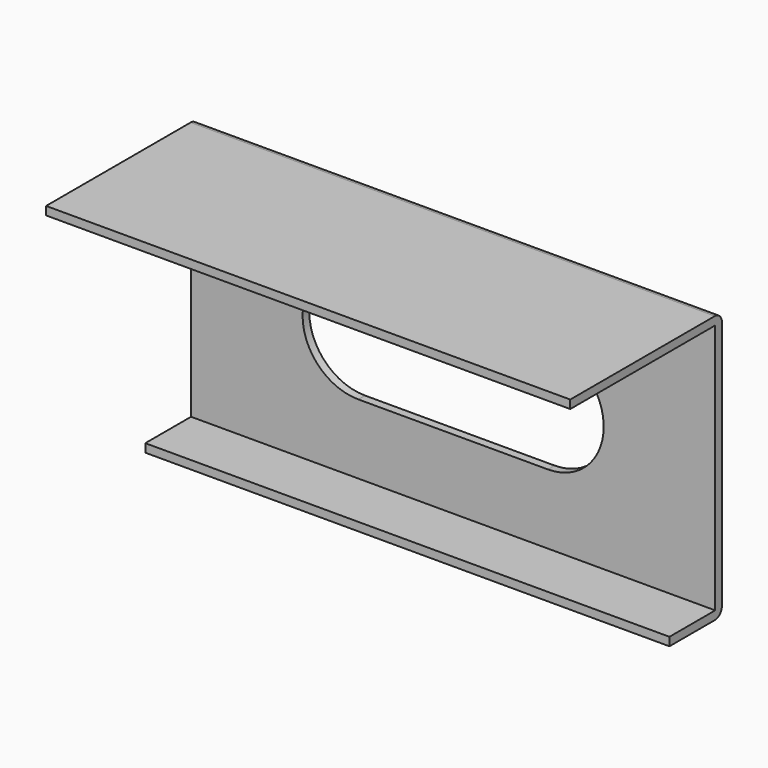
from build123d import *

# Parameters (mm, degrees)
F1_DEPTH = 298.45
F2_R     = 5.08
F4_D     = 63.5
F6_DEPTH = 25.4


with BuildPart() as f1:
    # F0 (on Right) → F1 (new body)
    with BuildSketch(Plane.YZ):
        Polygon((0, -85.7519404639), (0, 66.6480595361), (-107.95, 66.6480595361), (-107.95, 61.8728595361), (-4.7752, 61.8728595361), (-4.7752, -80.9767404639), (-37.338, -80.9767404639), (-37.338, -85.7519404639), align=None)
    extrude(amount=F1_DEPTH)

    # F2
    f2_edges = [f1.edges().sort_by_distance(p)[0] for p in [
        (149.225, 0, 66.64806),
        (149.225, 0, -85.75194),
    ]]
    fillet(f2_edges, radius=F2_R)

    # F4 (through all)
    with Locations(Plane(origin=(0, 0, 0), x_dir=(-1, 0, 0), z_dir=(0, 1, 0))):
        with Locations((-203.2, -9.5519404639), (-95.25, -9.5519404639)):
            Hole(F4_D / 2)

    # F5 (on face) → F6 (cut)
    with BuildSketch(Plane(origin=(0, 0, 0), x_dir=(-1, 0, 0), z_dir=(0, 1, 0))):
        with BuildLine():
            Line((-95.2632086497, 22.1980567886), (-201.5250755989, 22.1538496737))
            ThreePointArc((-201.5250755989, 22.1538496737), (-180.1647948812, 12.2985017543), (-171.45, -9.5519404639))
            ThreePointArc((-171.45, -9.5519404639), (-180.7493594116, -32.0025804808), (-203.1999991918, -41.3019404639))
            Line((-203.1999991918, -41.3019404639), (-95.2632086497, -41.3019377164))
            ThreePointArc((-95.2632086497, -41.3019377164), (-127, -9.5519404639), (-95.2632086497, 22.1980567886))
        make_face()
    extrude(amount=-F6_DEPTH, mode=Mode.SUBTRACT)


solid = f1.part
